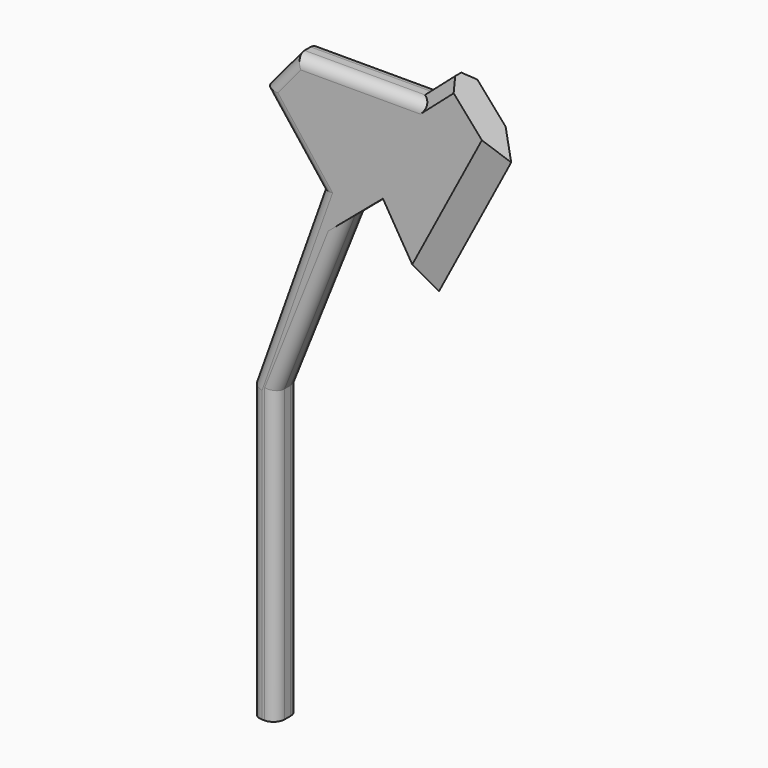
from build123d import *

# Parameters (mm, degrees)
F1_DEPTH    = 13.64111
F2_T1_DEPTH = 137.0825914491
F3_R        = 5.08
F4_SIZE     = 5.08
F5_R        = 5.08


# Not quite as in the source:
# - a fillet or chamfer that OpenCascade refuses, or shapes differently, is made with other operations: its cross-section is extruded or revolved along the edge and cut away or added


with BuildPart() as f1:
    # F0 (on Front) → F1 (new body)
    with BuildSketch(Plane.XZ):
        Polygon((0, 0), (16.8357715011, 14.2703205347), (38.0007438362, -20.6839479506), (71.29599154, 42.4681007862), (46.0088496082, 71.3043088503), (32.1346404756, 59.1376919794), (-23.249398917, 59.1376919794), (-38.0007401109, 41.5282361209), (-12.0255500078, 8.1773754209), (-43.7860488892, -80.4887861013), (-32.4603319168, -80.8862298727), align=None)
        Polygon((-32.4603319168, -214.6375030279), (-32.4603319168, -80.8862298727), (-43.7860488892, -80.4887861013), (-43.7860488892, -214.6375030279), align=None)
    extrude(amount=F1_DEPTH)

    # F2: chamfer of 7.62 x 12.7 on 2 edges, made by hand

    # F2_s2 → F2_t1 (cut)
    with BuildSketch(Plane(origin=(-15.5861012637, 0, -29.5626041102), x_dir=(0, 1, 0), z_dir=(0.4663751275, 0, 0.8845870451))):
        Polygon((-6.02111, -43.2614445663), (-13.64111, -30.5614445663), (-13.64111, -43.2614445663), align=None)
        Polygon((-7.62, -43.2614445663), (0, -30.5614445663), (0, -43.2614445663), align=None)
    extrude(amount=F2_T1_DEPTH, mode=Mode.SUBTRACT)

    # F3
    f3_edges = [f1.edges().sort_by_distance(p)[0] for p in [
        (-32.460332, -13.64111, -147.761866),
        (-32.460332, 0, -147.761866),
        (-43.786049, -13.64111, -147.563145),
        (-43.786049, 0, -147.563145),
        (-16.230166, -13.64111, -40.443115),
        (-27.905799, -13.64111, -36.155705),
        (-27.905799, 0, -36.155705),
        (-16.230166, 0, -40.443115),
    ]]
    fillet(f3_edges, radius=F3_R)

    # F4
    f4_edges = [f1.edges().sort_by_distance(p)[0] for p in [
        (39.071745, -13.64111, 65.221),
        (39.071745, 0, 65.221),
    ]]
    chamfer(f4_edges, length=F4_SIZE)

    # F5
    f5_edges = [f1.edges().sort_by_distance(p)[0] for p in [
        (-30.62507, -13.64111, 50.332964),
        (-30.62507, 0, 50.332964),
        (-25.013145, 0, 24.852806),
        (-25.013145, -13.64111, 24.852806),
        (4.442621, -13.64111, 59.137692),
        (4.442621, 0, 59.137692),
    ]]
    fillet(f5_edges, radius=F5_R)


solid = f1.part
